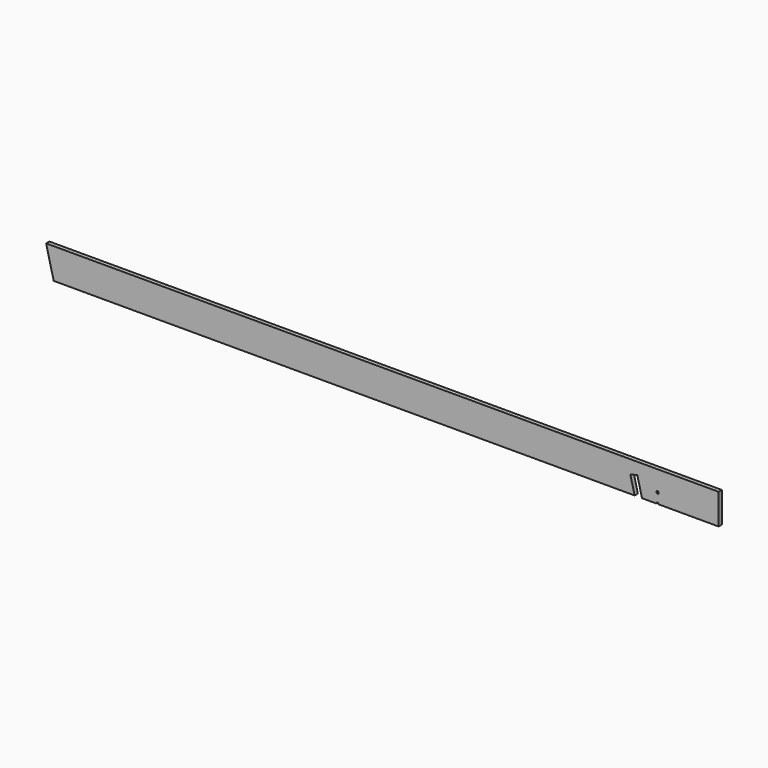
from build123d import *

# Parameters (mm, degrees)
F0_W        = 20
F0_H        = 150
F3_T1_DEPTH = 799.1426747922
F11_D       = 12


# Not quite as in the source:
# - a fillet or chamfer that OpenCascade refuses, or shapes differently, is made with other operations: its cross-section is extruded or revolved along the edge and cut away or added
# - a feature of the source that left no trace in its solid (it failed there, or was rolled back) is left out


with BuildPart() as f2:
    # F2: sweep along a path in F1
    with BuildLine(Plane.XZ) as f2_path:
        Line((0, 0), (-3300, 0))
    # F0 (on Right) → F2 (sweep)
    with BuildSketch(Plane.YZ):
        with Locations((-10, 75)):
            Rectangle(F0_W, F0_H)
    sweep(path=f2_path.line)

    # F3: chamfer of 150 x 37.3992004265 on 1 edges, made by hand

    # F3_s2 → F3_t1 (cut)
    with BuildSketch(Plane.XZ.offset(-389.5713373961)):
        Polygon((-3262.6007995735, 0), (-3300, 150), (-3300, 0), align=None)
    extrude(amount=F3_T1_DEPTH, mode=Mode.SUBTRACT)

    # F9: sweep along a path in F8
    with BuildLine(Plane.XY) as f9_path:
        Line((-375.5503296852, 160.6018841267), (-375.5503296852, -268.9945995808))
    # F7 (on Front) → F9 (sweep, cut)
    with BuildSketch(Plane.XZ):
        Polygon((-399.247874902, 92.5443589414), (-433.2082253216, 84.0770925954), (-352.1368366165, -241.0824874784), (-362.959590562, -53), align=None)
    sweep(path=f9_path.line, mode=Mode.SUBTRACT)

    # F11 (through all)
    with Locations(Plane(origin=(0, 0, 0), x_dir=(1, 0, 0), z_dir=(0, 1, 0))):
        with Locations((-300, -50), (-300, 0)):
            Hole(F11_D / 2)


solid = f2.part
